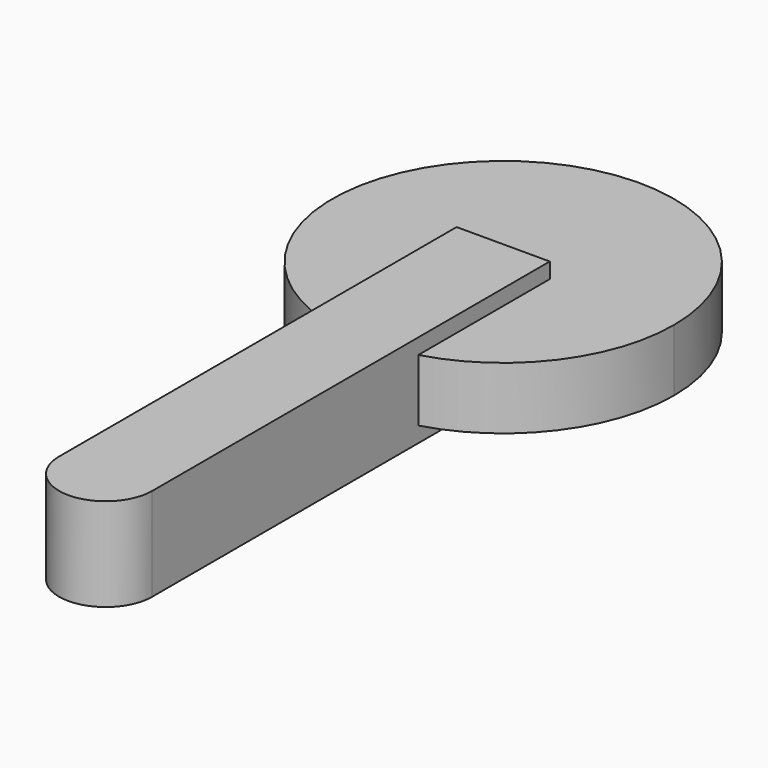
from build123d import *

# Parameters (mm, degrees)
F1_DEPTH = 6.35
F2_DEPTH = 7.9375
F3_DEPTH = 1.5875


# Not quite as in the source:
# - a length typed as a fraction of an inch, garbled in the dataset ("3 / 203.2 mm" for 3/8 in), is restored


with BuildPart() as f1:
    # F0 (on Top) → F1 (new body)
    with BuildSketch(Plane.XY):
        with BuildLine():
            ThreePointArc((-24.0030003875, -9.8155226706), (-14.8352444226, -3.5452855547), (-11.3030003875, 6.9849981546))
            ThreePointArc((-11.3030003875, 6.9849981546), (-39.2957840969, 20.9152541196), (-33.5280003875, -9.8155226706))
            Line((-33.5280003875, -9.8155226706), (-33.5280003875, 6.9849981546))
            Line((-33.5280003875, 6.9849981546), (-24.0030003875, 6.9849981546))
            Line((-24.0030003875, 6.9849981546), (-24.0030003875, -9.8155226706))
        make_face()
    extrude(amount=F1_DEPTH)

    # F0 (on Top) → F2 (join)
    with BuildSketch(Plane.XY):
        with BuildLine():
            Line((-33.5280003875, 6.9849981546), (-33.5280003875, -9.8155226706))
            ThreePointArc((-33.5280003875, -9.8155226706), (-28.7655003875, -10.4775018454), (-24.0030003875, -9.8155226706))
            Line((-24.0030003875, -9.8155226706), (-24.0030003875, 6.9849981546))
            Line((-24.0030003875, 6.9849981546), (-33.5280003875, 6.9849981546))
        make_face()
        with BuildLine():
            ThreePointArc((-24.0030003875, -9.8155226706), (-28.7655003875, -10.4775018454), (-33.5280003875, -9.8155226706))
            Line((-33.5280003875, -9.8155226706), (-33.5280003875, -43.8150018454))
            ThreePointArc((-33.5280003875, -43.8150018454), (-28.7655003875, -48.5775018454), (-24.0030003875, -43.8150018454))
            Line((-24.0030003875, -43.8150018454), (-24.0030003875, -9.8155226706))
        make_face()
    extrude(amount=F2_DEPTH)

    # F0 (on Top) → F3 (join)
    with BuildSketch(Plane.XY):
        with BuildLine():
            ThreePointArc((-24.0030003875, -9.8155226706), (-28.7655003875, -10.4775018454), (-33.5280003875, -9.8155226706))
            Line((-33.5280003875, -9.8155226706), (-33.5280003875, -43.8150018454))
            ThreePointArc((-33.5280003875, -43.8150018454), (-28.7655003875, -48.5775018454), (-24.0030003875, -43.8150018454))
            Line((-24.0030003875, -43.8150018454), (-24.0030003875, -9.8155226706))
        make_face()
        with BuildLine():
            Line((-33.5280003875, 6.9849981546), (-33.5280003875, -9.8155226706))
            ThreePointArc((-33.5280003875, -9.8155226706), (-28.7655003875, -10.4775018454), (-24.0030003875, -9.8155226706))
            Line((-24.0030003875, -9.8155226706), (-24.0030003875, 6.9849981546))
            Line((-24.0030003875, 6.9849981546), (-33.5280003875, 6.9849981546))
        make_face()
    extrude(amount=-F3_DEPTH)


solid = f1.part
